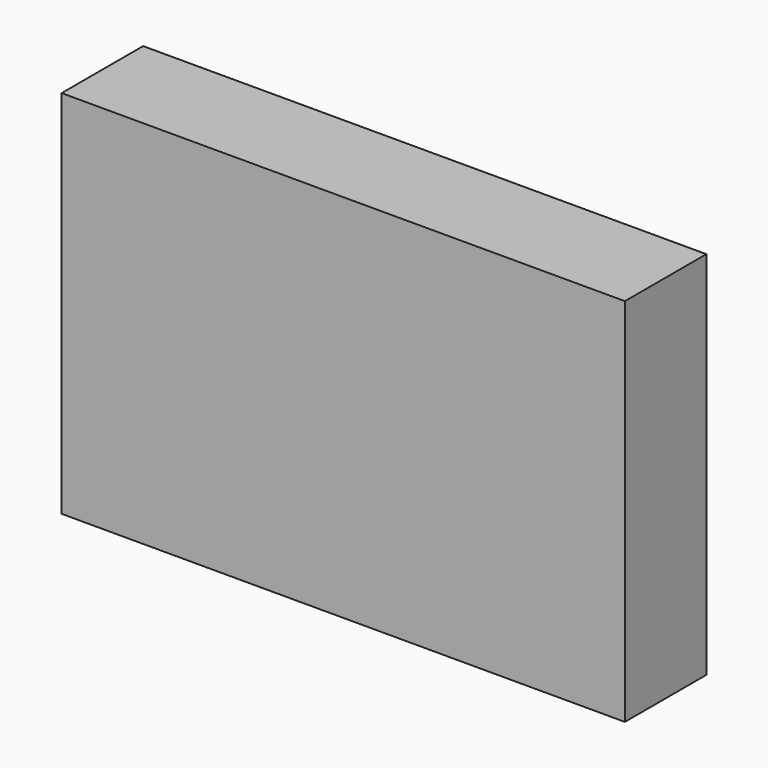
from build123d import *

# Parameters (mm, degrees)
F0_W     = 140.5029818416
F0_H     = 92.4022980034
F1_DEPTH = 25.4


# Not quite as in the source:
# - the program builds the solid bodies; features that only make, move or delete a surface that nothing else refers to are left out


with BuildPart() as f1:
    # F0 (on Front) → F1 (new body)
    with BuildSketch(Plane.XZ):
        with Locations((11.3195665181, 24.2008250207)):
            Rectangle(F0_W, F0_H)
    extrude(amount=F1_DEPTH)


solid = f1.part
